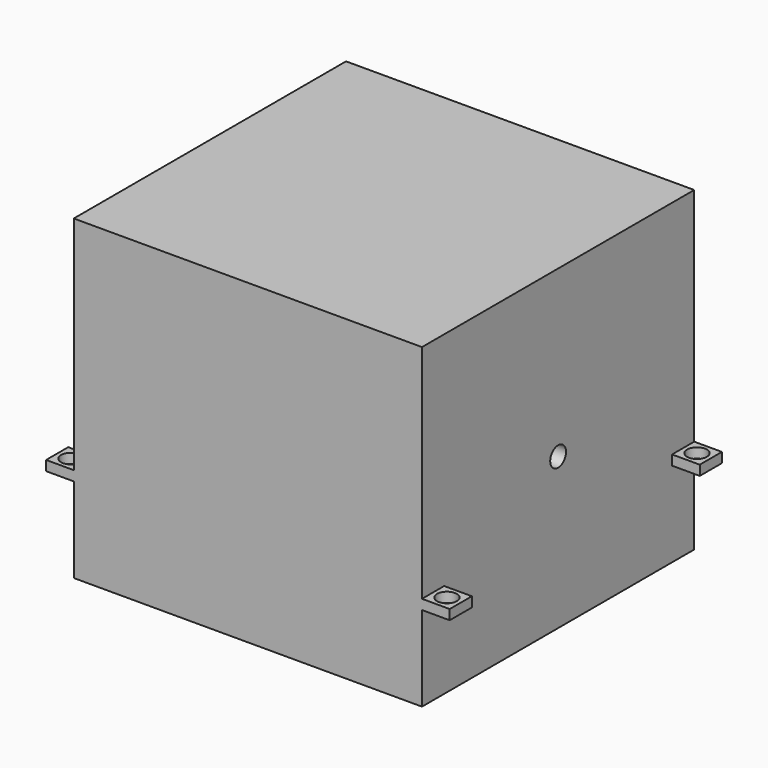
from build123d import *

# Parameters (mm, degrees)
F1_DEPTH  = 80
F8_DEPTH  = 2.5
F9_T      = -4
F10_D     = 5
F14_D     = 5
F15_D     = 5
F15_DEPTH = 51.001


with BuildPart() as f1:
    # F0 (on Top) → F1 (new body)
    with BuildSketch(Plane.XY):
        Polygon((44, -43), (44, 43), (37, 43), (-37, 43), (-44, 43), (-44, -43), (-37, -43), (37, -43), align=None)
    extrude(amount=F1_DEPTH)

    # F7 (on 3pt) → F8 (join)
    with BuildSketch(Plane.XY.offset(21.5)):
        Polygon((-47.5, 39.5), (-51, 43), (-51, 36), align=None)
        Polygon((-51, 36), (-44, 36), (-47.5, 39.5), align=None)
        Polygon((-44, 36), (-44, 43), (-47.5, 39.5), align=None)
        Polygon((-47.5, 39.5), (-44, 43), (-51, 43), align=None)
        Polygon((51, 43), (44, 43), (47.5, 39.5), align=None)
        Polygon((47.5, 39.5), (44, 36), (51, 36), align=None)
        Polygon((51, 36), (51, 43), (47.5, 39.5), align=None)
        Polygon((47.5, 39.5), (44, 43), (44, 36), align=None)
        Polygon((47.5, -39.5), (44, -43), (51, -43), align=None)
        Polygon((51, -36), (44, -36), (47.5, -39.5), align=None)
        Polygon((51, -43), (51, -36), (47.5, -39.5), align=None)
        Polygon((47.5, -39.5), (44, -36), (44, -43), align=None)
        Polygon((-44, -43), (-44, -36), (-47.5, -39.5), align=None)
        Polygon((-47.5, -39.5), (-44, -36), (-51, -36), align=None)
        Polygon((-51, -43), (-47.5, -39.5), (-51, -36), align=None)
        Polygon((-51, -43), (-44, -43), (-47.5, -39.5), align=None)
    extrude(amount=F8_DEPTH)

    # F9
    f9_openings = [f1.faces().sort_by_distance(p)[0] for p in [
        (0, 0, 0),
    ]]
    offset(amount=F9_T, openings=f9_openings, kind=Kind.INTERSECTION)

    # F10 (through all)
    with Locations(Plane(origin=(0, 0, 21.5), x_dir=(1, 0, 0), z_dir=(0, 0, -1))):
        with Locations((47.5, 39.5), (47.5, -39.5), (-47.5, -39.5), (-47.5, 39.5)):
            Hole(F10_D / 2)

    # F14 (through all)
    with Locations(Plane(origin=(44, 0, 0), x_dir=(0, -1, 0), z_dir=(1, 0, 0))):
        with Locations((0, -38.1846800447)):
            Hole(F14_D / 2)

    # F15 (through all, one way)
    with BuildSketch(Plane.YZ):
        with Locations((0, 38.2145792246)):
            Circle(F15_D / 2)
    extrude(amount=-F15_DEPTH, mode=Mode.SUBTRACT)


solid = f1.part
